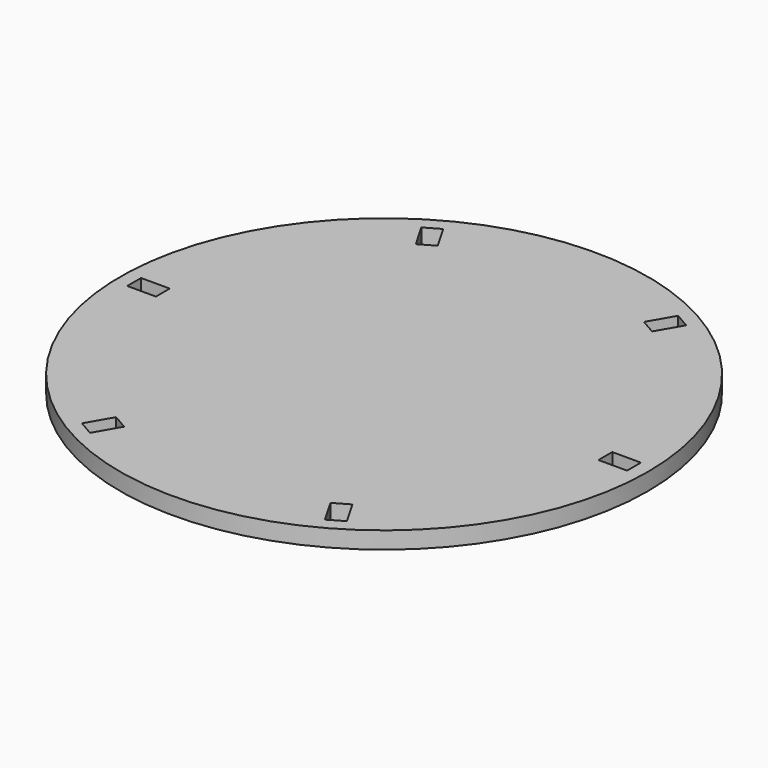
from build123d import *

# Parameters (mm, degrees)
F2_R     = 1181.8412542343
F2_W     = 128.27
F2_H     = 77.47
F3_DEPTH = 76.2


with BuildPart() as f3:
    # F2 (on face) → F3 (new body)
    with BuildSketch(Plane.XY.offset(-1151.068019867)):
        Circle(F2_R)
        Polygon((-525.9426331016, -988.4293623985), (-593.0336211327, -949.6943623985), (-528.8986211327, -838.609283855), (-461.8076331016, -877.344283855), align=None, mode=Mode.SUBTRACT)
        Polygon((593.0336211327, -949.6943623985), (525.9426331016, -988.4293623985), (461.8076331016, -877.344283855), (528.8986211327, -838.609283855), align=None, mode=Mode.SUBTRACT)
        with Locations((-1054.8412542343, 0)):
            Rectangle(F2_W, F2_H, mode=Mode.SUBTRACT)
        Polygon((-593.0336211327, 949.6943623985), (-525.9426331016, 988.4293623985), (-461.8076331016, 877.344283855), (-528.8986211327, 838.609283855), align=None, mode=Mode.SUBTRACT)
        with Locations((1054.8412542343, 0)):
            Rectangle(F2_W, F2_H, mode=Mode.SUBTRACT)
        Polygon((525.9426331016, 988.4293623985), (593.0336211327, 949.6943623985), (528.8986211327, 838.609283855), (461.8076331016, 877.344283855), align=None, mode=Mode.SUBTRACT)
    extrude(amount=-F3_DEPTH)


solid = f3.part
